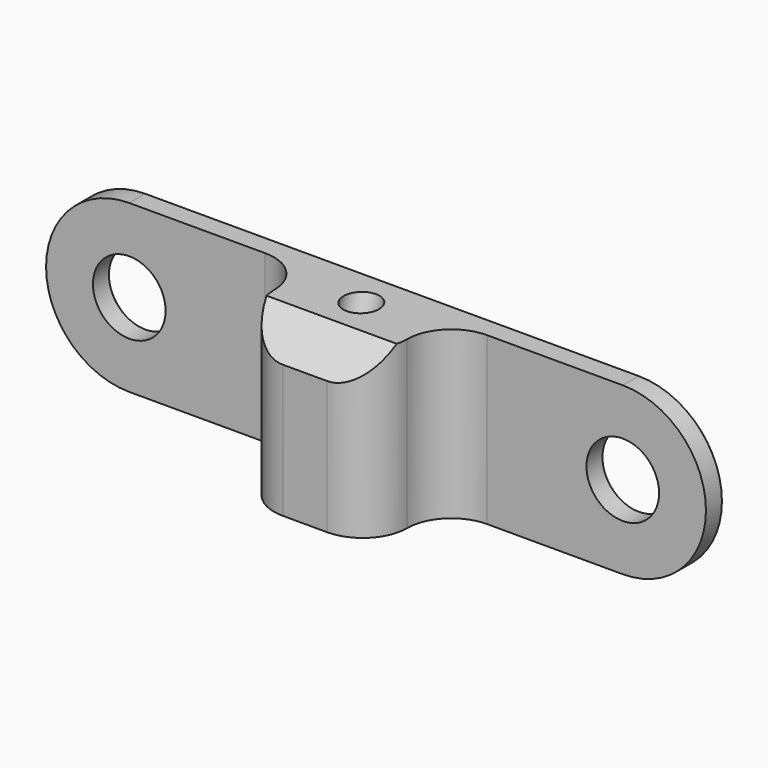
from build123d import *

# Parameters (mm, degrees)
F0_R         = 3.275
F1_DEPTH     = 2
F3_W         = 8
F3_H         = 15
F4_DEPTH     = 6
F5_SIZE      = 3
F6_R         = 3.99999
F8_SIZE      = 0.2
F9_TEXT_SIZE = 15.2824565798
F10_DEPTH    = 0.2


# Not quite as in the source:
# - a fillet or chamfer is up to 0.001 mm smaller than in the source, because OpenCascade refuses the exact size
# - Text() gives the source's letters only with a copy of the font that has no kerning and outlines rounded to 1/6400 em; it was checked with that copy


with BuildPart() as f1:
    # F0 (on Front) → F1 (new body)
    with BuildSketch(Plane.XZ):
        with BuildLine():
            ThreePointArc((-22.25, 7.5), (-29.75, 0), (-22.25, -7.5))
            Line((-22.25, -7.5), (22.25, -7.5))
            ThreePointArc((22.25, -7.5), (29.75, 0), (22.25, 7.5))
            Line((22.25, 7.5), (-22.25, 7.5))
        make_face()
        with Locations((-22.25, 0)):
            Circle(F0_R, mode=Mode.SUBTRACT)
        with Locations((22.25, 0)):
            Circle(F0_R, mode=Mode.SUBTRACT)
    extrude(amount=-F1_DEPTH)

    # F3 (on Right) → F4 (join, symmetric)
    with BuildSketch(Plane.YZ):
        with Locations((-4, 0)):
            Rectangle(F3_W, F3_H)
    extrude(amount=F4_DEPTH, both=True)

    # F5
    f5_edges = [f1.edges().sort_by_distance(p)[0] for p in [
        (0, -8, 7.5),
    ]]
    chamfer(f5_edges, length=F5_SIZE)

    # F6 (radius 4 in the source; OpenCascade refuses exactly that, so slightly less here)
    f6_edges = [f1.edges().sort_by_distance(p)[0] for p in [
        (6, 0, 0),
        (-6, 0, 0),
        (6, -8, -1.5),
        (-6, -8, -1.5),
    ]]
    fillet(f6_edges, radius=F6_R)

    # F2 (on Right) → F7 (revolve, cut)
    with BuildSketch(Plane.YZ):
        Polygon((-6.1967911854, -3.2628889711), (-4.6513098633, -3.6769994433), (7.335233061, 41.0573877571), (5.7897517389, 41.4714982292), align=None)
    revolve(axis=Axis((0, 1.3419615988, 18.6901941569), (0, -0.2588190451, -0.9659258263)), mode=Mode.SUBTRACT)

    # F8
    f8_edges = [f1.edges().sort_by_distance(p)[0] for p in [
        (-29.75, 2, 0),
        (0, 2, -7.5),
        (29.75, 2, 0),
        (0, 2, 7.5),
        (-25.525, 2, 0),
        (18.975, 2, 0),
    ]]
    chamfer(f8_edges, length=F8_SIZE)

    # F9 (on face) → F10 (cut)
    with BuildSketch(Plane(origin=(0, 2, 0), x_dir=(-1, 0, 0), z_dir=(0, 1, 0))):
        with Locations((-8.793382243, -5.5016843687)):
            Text('15', F9_TEXT_SIZE, font='Open Sans', text_align=(TextAlign.LEFT, TextAlign.BOTTOM))
    extrude(amount=-F10_DEPTH, mode=Mode.SUBTRACT)


solid = f1.part
